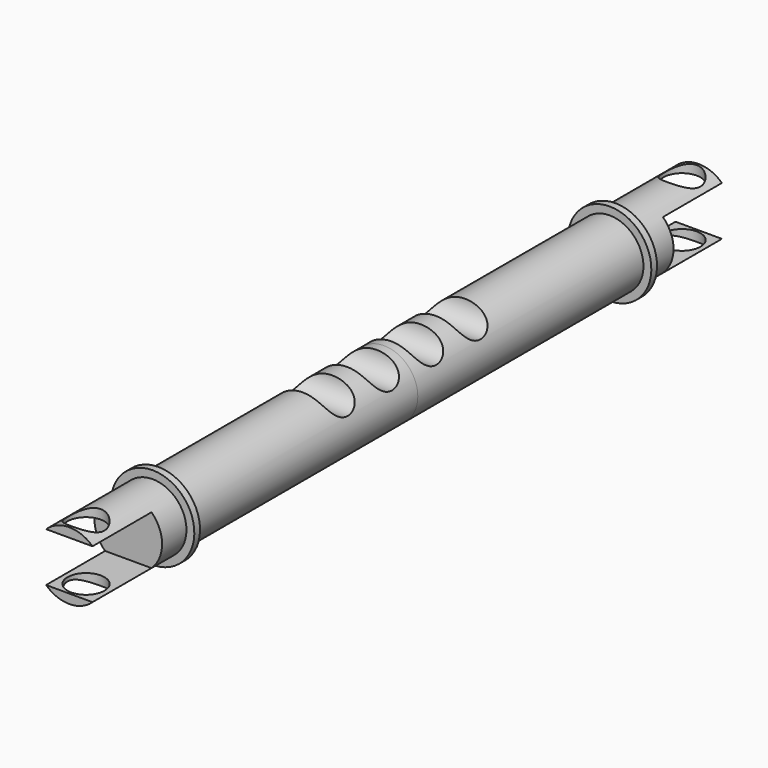
from build123d import *

# Parameters (mm, degrees)
F0_R     = 13.75
F1_DEPTH = 160
F3_DEPTH = 12.5
F4_W     = 37.5
F4_H     = 20
F5_DEPTH = 30
F6_R     = 7.5
F7_DEPTH = 1000
F2_W     = 2.9
F2_H     = 3.2


# Not quite as in the source:
# - a feature names something its author has since deleted; it is built from what else it names


with BuildPart() as f1:
    # F0 (on Front) → F1 (new body)
    with BuildSketch(Plane.XZ):
        Circle(F0_R)
    extrude(amount=F1_DEPTH)

    # F2 (on Right) → F3 (cut, symmetric)
    with BuildSketch(Plane.YZ):
        with BuildLine():
            Line((-141.25, 13.75), (-156.25, 13.75))
            ThreePointArc((-156.25, 13.75), (-148.75, 6.25), (-141.25, 13.75))
        make_face()
        with BuildLine():
            ThreePointArc((-133.75, 13.75), (-126.25, 6.25), (-118.75, 13.75))
            Line((-118.75, 13.75), (-133.75, 13.75))
        make_face()
    extrude(amount=F3_DEPTH, both=True, mode=Mode.SUBTRACT)

    # F4 (on Front) → F5 (cut)
    with BuildSketch(Plane.XZ):
        Rectangle(F4_W, F4_H)
    extrude(amount=F5_DEPTH, mode=Mode.SUBTRACT)

    # F6 (on Top) → F7 (cut, symmetric)
    with BuildSketch(Plane.XY):
        with Locations((0, -8.5)):
            Circle(F6_R)
    extrude(amount=F7_DEPTH, both=True, mode=Mode.SUBTRACT)

    # F2 (on Right) → F8 (revolve)
    with BuildSketch(Plane.YZ):
        with Locations((-43.8301734209, 15.35)):
            Rectangle(F2_W, F2_H)
    revolve(axis=Axis((0, -35.3111437289, 0), (0, -1, 0)))

    # F9: F1 across face


with BuildPart() as f1_1:
    add(f1.part)
    add(f1.part.mirror(Plane.XZ.offset(160)))


solid = f1_1.part
